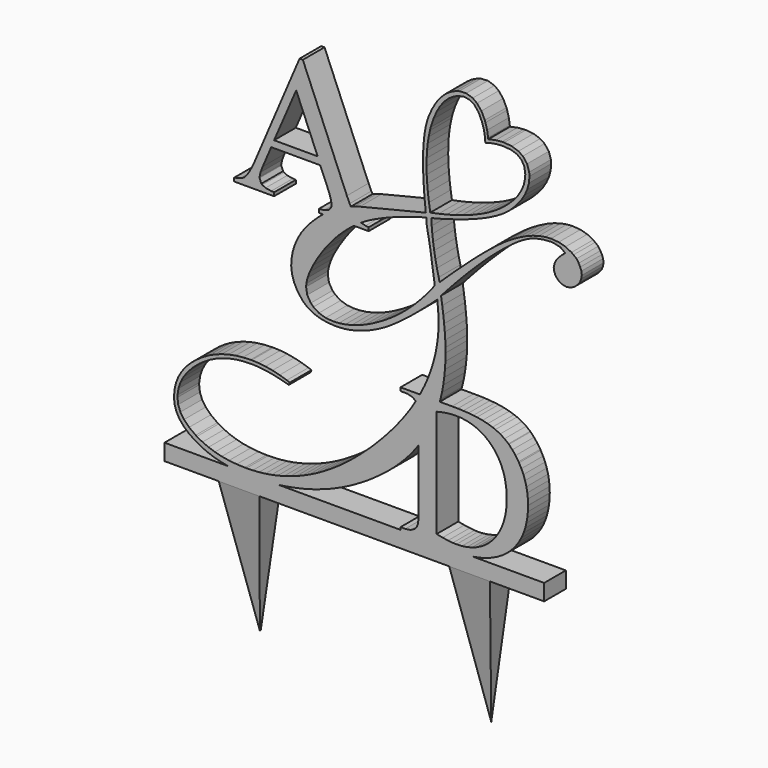
from build123d import *

# Parameters (mm, degrees)
F1_DEPTH = 10
F3_DEPTH = 10
F5_DEPTH = 140.001


# Not quite as in the source:
# - ends of sketch curves that miss each other by under 0.0002 mm in the source are joined


with BuildPart() as f1:
    # F0 (on Front) → F1 (new body)
    with BuildSketch(Plane.XZ):
        Polygon((-10.9298886665, 24.1676968787), (-9.9886611628, 24.5012024907), (-10.4234494528, 25.3038880581), (-11.4401839308, 27.5444704665), (-27.6891162725, 66.3875142995), (-30.1368107855, 55.6929674748), (-22.2288717636, 36.8268846491), (-38.2895193935, 36.8268846491), (-21.26862216, 34.2473902988), (-18.4443582236, 27.5444704665), (-17.8795054363, 26.0946816908), (-17.2769965153, 24.1741824836), (-17.0698830629, 22.7432224485), (-17.2769965153, 21.7076592298), (-18.067790148, 20.8415506343), (-19.5175789237, 20.2202129726), (-19.8564908657, 20.1260706168), (-21.8146462065, 19.9189585121), (-21.8146462065, 18.6386257073), (-20.2368925623, 18.6386257073), (-19.9110483886, 18.9145658222), (-17.7457782476, 20.4961530874), (-15.5428533206, 21.9082857296), (-13.2646134308, 23.13213366), align=None)
        Polygon((-30.1368107855, 55.6929674748), (-27.6891162725, 66.3875142995), (-28.8941354622, 66.3875142995), (-45.2936936863, 27.9586960236), (-45.3690073014, 27.7704126597), (-46.4045705201, 25.5298289035), (-47.3836488644, 23.7034720521), (-48.3250710751, 22.2725120171), (-49.1911783228, 21.2557761913), (-49.3229768124, 21.1428064425), (-50.697451973, 20.4649825587), (-52.9945206036, 19.9189585121), (-52.9945206036, 18.6386257073), (-38.2895193935, 18.6386257073), (-38.2895193935, 19.9189585121), (-39.343911353, 19.9942721272), (-41.4150377904, 20.3331840692), (-42.6577144615, 20.9168655972), (-42.9777976627, 21.1992913169), (-43.6556215466, 22.8373648044), (-43.6556215466, 23.1197905241), (-43.3167096047, 24.7578640116), (-42.5070872313, 26.8666479305), (-39.343911353, 34.2473902988), (-21.26862216, 34.2473902988), (-38.2895193935, 36.8268846491), align=None)
        Polygon((-10.1767511675, -15.6167678171), (-7.6537430394, -15.0330862891), (-16.6349014137, -14.8636303181), (-19.3085381199, -14.6376894728), (-21.7562339807, -13.8657232331), (-23.7897042845, -12.5665630354), (-24.7499538881, -11.6251408247), (-26.0491140858, -9.4410432907), (-26.4821683836, -6.9368625555), (-26.3880260277, -5.788329588), (-25.9549730778, -3.8301728993), (-25.1453507044, -1.6272466246), (-23.9591589076, 0.8392766292), (-22.3964003831, 3.5505708168), (-20.4570724352, 6.487804502), (-19.7604198106, 7.485711587), (-18.0846901895, 9.669809121), (-16.3336469532, 11.7409355585), (-14.5072901019, 13.6990922471), (-12.6056182876, 15.5254490985), (-10.6474629468, 17.2388362011), (-8.885374772, 18.6386257073), (-20.2368925623, 18.6386257073), (-22.0010035668, 17.1446938452), (-24.0533012635, 15.1865371566), (-24.8817523776, 14.3204299088), (-26.7645954511, 12.1551611155), (-28.3650114571, 9.9334061001), (-29.6641730027, 7.655167558), (-30.6620787399, 5.3580989274), (-31.3963874982, 3.0045454224), (-31.8294417959, 0.6133357838), (-31.9800690262, -1.8155313363), (-31.9612402854, -2.0603009224), (-31.6788145657, -4.5268241761), (-30.9256770667, -6.9180351625), (-29.7018291363, -9.2715873197), (-28.0072707745, -11.5309984688), (-27.5177316023, -12.0770238632), (-25.7666883661, -13.5456400319), (-23.6767331879, -14.6753456065), (-21.2666948085, -15.4849679798), (-18.536573228, -15.974507152), (-15.4675397055, -16.1439631229), (-15.0909702821, -16.1439631229), (-12.6432757691, -15.9933358927), align=None)
        Polygon((-9.4443711085, 23.4963599475), (-9.9886611628, 24.5012024907), (-10.9298886665, 24.1676968787), (-13.2646134308, 23.13213366), (-15.5428533206, 21.9082857296), (-17.7457782476, 20.4961530874), (-19.9110483886, 18.9145658222), (-20.2368925623, 18.6386257073), (-8.885374772, 18.6386257073), (-8.6328213837, 18.8392522071), (-6.5240374648, 20.3078697236), (-6.1985443859, 20.5113026795), (-6.4318224604, 20.5779536553), (-7.8627838432, 21.4628896437), (-8.5029502456, 22.1407121798), align=None)
        Polygon((14.6391139914, 29.100744734), (17.8964308778, 30.0421655968), (17.6751323737, 31.5131313185), (-6.6558359543, 25.5610007801), (-8.5386790279, 25.0149753857), (-9.9886611628, 24.5012024907), (-9.4443711085, 23.4963599475), (-8.5029502456, 22.1407121798), (-7.8627838432, 21.4628896437), (-6.4318224604, 20.5779536553), (-6.1985443859, 20.5113026795), (-5.0177624669, 21.2492905864), (-3.1914056155, 22.2660250644), (-1.1767640525, 23.2639321495), (1.0073334815, 24.2618392345), (3.3797143794, 25.2597449718), (5.9215525961, 26.2388233161), (8.6516741767, 27.1990729197), (11.5512517282, 28.1593225233), align=None)
        Polygon((19.3254703004, 30.5748801363), (19.3520434895, 30.3486104282), (19.6851315955, 30.4187336724), (23.0742483192, 31.3036696609), (26.4068801685, 32.2450918716), (29.5512273061, 33.2053414752), (32.4884609913, 34.1655910788), (35.2185839196, 35.1446694231), (37.7604207885, 36.1425751604), (40.0951455527, 37.1593109862), (42.2227582124, 38.1948742049), (44.1432574196, 39.2304374236), (45.8754719151, 40.284829383), (47.4005743059, 41.3580500832), (48.7185645922, 42.4312694356), (50.8838333855, 44.6153669696), (52.6913628439, 46.7994645036), (54.0846667453, 49.0212195191), (55.0825724825, 51.2429731867), (55.6850827513, 53.4835555951), (55.8733661152, 55.7429667443), (55.7792251071, 57.0986131642), (55.0072588674, 59.5274802843), (53.4444989951, 61.5044657137), (51.8064268554, 62.577685066), (46.1578989826, 62.3894017021), (49.0574765341, 62.1446321161), (51.3733725576, 61.3726658764), (53.0114460451, 60.0546769379), (54.0093517824, 58.2283187387), (54.3482637243, 55.8747665816), (54.2352939755, 54.3496628429), (53.7645835441, 52.2032227903), (52.8608188149, 50.0944388714), (51.5804860101, 48.0044836933), (49.8670989075, 45.9521859966), (47.7771437293, 43.9375444335), (45.2729629941, 41.9229028705), (44.2750559091, 41.2450789866), (42.3922141833, 40.040059797), (40.3775726203, 38.9103542224), (38.2123024792, 37.8371335222), (35.9152351964, 36.839227785), (33.4863680763, 35.8789781814), (30.9257024667, 34.9940421929), (28.2144082791, 34.1844198195), (25.3901443427, 33.4124535798), (22.415253176, 32.715802303), (19.3085635199, 32.0756359006), align=None)
        Polygon((19.3085635199, 32.0756359006), (17.8964308778, 30.0421655968), (19.3520435853, 30.3486099733), (19.3254703004, 30.5748801363), align=None)
        Polygon((17.6751323737, 31.5131313185), (17.8964308778, 30.0421655968), (19.3085635199, 32.0756359006), (17.8964308778, 31.5672679877), align=None)
        Polygon((17.8964308778, 31.5672679877), (19.3085635199, 32.0756359006), (18.8232483473, 35.2102505875), (18.4368979524, 38.2410969438), (18.1737322688, 41.1571122421), (17.9853100817, 43.980424633), (17.9200726059, 46.688904618), (17.9714412383, 49.3001948754), (18.1041319702, 51.801140895), (18.3534301582, 54.204897187), (18.7082690314, 56.4872438179), (19.1797140128, 58.6723993735), (19.466277473, 59.8442115114), (20.4793176362, 62.8943677724), (21.6370452829, 65.5563891538), (22.9615912596, 67.8787155224), (24.4726886794, 69.8084188435), (26.1329617509, 71.3918485489), (27.97978357, 72.5826565544), (29.3693621572, 73.221225816), (31.6930511498, 73.7257511562), (33.7529356025, 73.4286411752), (35.5600822863, 72.354118502), (37.0923590069, 70.453740574), (38.3345262104, 67.8222993858), (36.5379354821, 73.1808040004), (34.9601409209, 74.3408255997), (32.5618149078, 75.1145938456), (30.0162918109, 74.9895383904), (28.7131515651, 74.604227148), (26.6618229353, 73.638597134), (24.7728258152, 72.2914081477), (23.0395816019, 70.5803055631), (21.444447617, 68.4987107771), (20.0292878202, 66.0421356218), (18.7390837414, 63.2503536218), (18.1938346788, 61.6405084197), (17.7209286841, 59.8365964516), (17.3380084357, 57.845193625), (17.0384980261, 55.6839426181), (16.8113320322, 53.3286261931), (16.6741517845, 50.7858175617), (16.6269586308, 48.0555194196), (16.6631739682, 45.1553730972), (16.7893763996, 42.0677372641), (16.9879232467, 38.7860333172), (17.2698785849, 35.334482538), (17.6244923758, 31.8497341414), (17.6751323737, 31.5131313185), align=None)
        Polygon((46.1578989826, 62.3894017021), (51.8064268554, 62.577685066), (49.3963884761, 63.4061361801), (46.5344670582, 63.6697345069), (45.7625021663, 63.6509057662), (43.4466061428, 63.4437936616), (41.1307087715, 62.9542544894), (40.6390589473, 62.8273781589), (40.6869516082, 61.630595364), (41.3943070983, 61.8433776556), (43.7478606032, 62.2576018648), align=None)
        Polygon((36.5379354821, 73.1808040004), (38.3345262104, 67.8222993858), (39.0528487343, 65.5180267738), (39.486804709, 63.1680314561), (39.6073046063, 61.3058231729), (40.686951551, 61.6305955543), (40.639059768, 62.8273781917), (40.6197840854, 63.309063711), (40.2695506387, 65.650081345), (39.6546824083, 67.8924468904), (39.4026791893, 68.6223645222), (38.1560238179, 71.2119444463), align=None)
        Polygon((16.1642163823, -26.9138235628), (15.4680634141, -28.2097382624), (22.7963671558, -28.2097382624), (23.0365921855, -27.3657052535), (23.6202723657, -24.880353259), (24.090984145, -22.3385150423), (24.4487234798, -19.759020692), (24.7123218066, -17.1042127265), (24.8817777776, -14.4117486274), (24.938262652, -11.6627983062), (24.9006065183, -9.8740975885), (24.8252915554, -7.4828879498), (24.6558369322, -4.9598784739), (24.4110673462, -2.3238992492), (24.1098115379, 0.4438798128), (23.7144147216, 3.3434573644), (23.2625330309, 6.3748347532), (24.9570913927, 8.2576764789), (26.8964193406, 10.4041178793), (22.754165118, 10.5924012432), (22.3964257831, 12.0798475004), (21.7562593807, 14.8476252146), (21.2102339864, 17.577748143), (20.7395235549, 20.2325561084), (20.3629554793, 22.8497065924), (20.0617010189, 25.4292009427), (19.8357588257, 27.9522104187), (19.6851315955, 30.4187336724), (19.3520435853, 30.3486099733), (17.8964308778, 30.0421655968), (18.0282307151, 27.0861031709), (18.1788579453, 26.5212503837), (18.630739636, 24.2430104938), (19.3085635199, 20.3078697236), (20.9654644003, 8.9355003628), (19.7416178177, 7.3539117497), (17.9529171, 5.1698142157), (21.8692291295, 4.6991037843), (22.0951699748, 2.5714924725), (22.3022834273, -0.1586291081), (22.3775970424, -2.4556977387), (22.3399395609, -4.0561137447), (22.2269698121, -6.3531823753), (21.9822002261, -8.6502496581), (21.6244595434, -10.9284895479), (21.1725778527, -13.2255568307), (20.6077250654, -15.5037967205), (19.9299011816, -17.8008653511), (19.1579362897, -20.0791038932), (18.2730003012, -22.357343783), (17.2750932161, -24.6355836729), align=None)
        Polygon((19.2897347792, 2.3455516271), (21.8692291295, 4.6991037843), (17.9529171, 5.1698142157), (16.1265589008, 3.117516519), (14.2437171751, 1.1405310896), (12.3420453608, -0.7234818954), (10.38389002, -2.4745264794), (8.3880758498, -4.1314273598), (6.3546068939, -5.6753584914), (4.2834791086, -7.1251472672), (2.1746951897, -8.4619649464), (0.4989655686, -9.4598720314), (-2.1370136561, -10.8908320664), (-4.7165080064, -12.1146799969), (-7.2395174823, -13.0937583412), (-9.6872119954, -13.8657232331), (-12.0595942411, -14.4305760204), (-14.3754902646, -14.7506592216), (-16.6349014137, -14.8636303181), (-7.6537430394, -15.0330862891), (-5.1119048227, -14.2234639157), (-2.5135817317, -13.187900697), (0.122397493, -11.9263952852), (0.6119366652, -11.6816256991), (2.2876662863, -10.7590335769), (4.0575382633, -9.666984136), (5.9215525961, -8.4243088127), (7.8985366777, -7.0310049113), (9.9696644629, -5.4682463868), (12.1537619969, -3.7548592842), (14.432000539, -1.8720162107), (16.8043827847, 0.1614540931), align=None)
        Polygon((22.754165118, 10.5924012432), (26.8964193406, 10.4041178793), (28.8169185478, 12.4752443167), (30.7185890143, 14.4898858798), (32.6014320878, 16.4292138277), (34.4654464206, 18.3120555534), (36.291803272, 20.1195850119), (38.1181614712, 21.8706282481), (39.906860841, 23.5651866099), (41.676732818, 25.1656026159), (42.2039294716, 25.6363143952), (44.8587374371, 27.9145529372), (47.3064332979, 29.9103671073), (49.5281869656, 31.6237528621), (51.5239997879, 33.0358855042), (53.2938717648, 34.1655910788), (54.8566316372, 35.0128695858), (56.0804795676, 35.5588949802), (58.6223164365, 36.4061734872), (61.1829833939, 36.8957126593), (63.8001338778, 37.0651686303), (69.1850634238, 37.1969671198), (66.6620552957, 37.8747910037), (63.8001338778, 38.100731849), (61.6725212182, 37.9501046188), (59.3754539354, 37.5358790617), (56.9654155561, 36.8203990442), (54.4612348209, 35.8224919592), (51.8252555961, 34.5421591544), (49.0951326678, 32.9794006298), (47.7771437293, 32.132120775), (46.3085262128, 31.13421369), (44.7269389476, 29.9856807225), (43.0323805857, 28.6865191769), (41.2248511273, 27.2555591419), (39.3231806608, 25.6739705288), (37.2897103571, 23.9605834263), (35.1432689567, 22.0965704412), (32.9026865483, 20.0819288782), (30.5303056504, 17.9166587371), (28.0449536559, 15.6195914543), (25.4654593056, 13.1718955935), align=None)
        Polygon((69.1850634238, 37.1969671198), (63.8001338778, 37.0651686303), (64.5909275105, 37.0275111489), (67.2645642166, 36.4250022279), (69.0532649343, 35.1446694231), (69.0344361936, 35.0505270673), (67.9642696041, 34.1886222543), (67.0009658898, 33.2241702159), (66.247446964, 32.4437330646), (65.6371720299, 31.5799359429), (65.1351333773, 30.4364666532), (64.8356970966, 29.1384008676), (64.9674969339, 27.8957255443), (65.4550750597, 26.7201368759), (66.2290009979, 25.6927992696), (67.1139369864, 24.977319252), (68.2955651385, 24.5026826845), (69.5616328472, 24.2806666275), (71.1620488532, 24.563093695), (72.3996308472, 25.2280824967), (73.4026312616, 26.0693673451), (74.5511655769, 27.500328728), (74.971341663, 28.6815458016), (75.1913319793, 29.9103671073), (75.0407047491, 31.2283560458), (74.581185086, 32.3683803633), (74.042797664, 33.4501110613), (73.2342090519, 34.6332703121), (72.1222984568, 35.5400662394), (71.3691609579, 36.086090286), align=None)
        Polygon((14.9403684519, -29.1920621048), (13.9460917161, -30.8965359279), (14.0773234016, -30.9963460652), (14.6045200552, -32.0507380246), (14.9246032564, -33.877094876), (15.0375730052, -36.4565892263), (15.0375730052, -44.7636998826), (16.013589152, -43.3322105276), (17.3315780905, -41.204597868), (18.5554260209, -39.0393290747), (19.6663028547, -36.7987466663), (20.6642099398, -34.5205067764), (21.5491459283, -32.1857820122), (21.6463504816, -31.8941683522), (21.6463504816, -31.7871396978), (21.6850938894, -31.777938129), (22.3399395609, -29.8134011143), (22.7963671558, -28.2097382624), (15.4680634141, -28.2097382624), align=None)
        Polygon((12.7405057224, -29.9796102394), (13.9460917161, -30.8965359279), (14.9403684519, -29.1920621048), (15.4680634141, -28.2097382624), (8.3346545207, -28.2097382624), (8.3346545207, -29.4524149336), (10.085697757, -29.4524149336), (10.8953201303, -29.4900710672), align=None)
        Polygon((-48.4737696061, -72.9304963116), (-60.4674779763, -73.2317507721), (-58.0009533748, -73.9095746559), (-55.3838028908, -74.4367699617), (-52.6536799624, -74.8133380373), (-49.7917598924, -75.0392802305), (-46.798039985, -75.1145938456), (-45.5553646617, -75.0957651049), (-42.9005553484, -75.0204514898), (-40.2645761237, -74.8509955188), (-37.6474256397, -74.6062259327), (-35.0679312894, -74.2861427315), (-32.507264332, -73.8530884337), (-29.9654274631, -73.3635492616), (-27.4612467279, -72.7798690814), (-24.9758947334, -72.1208739382), (-22.5281988726, -71.3677364392), (-20.0993317525, -70.5204579322), (-17.6892933732, -69.616693203), (-15.3169124753, -68.618786118), (-12.9445302296, -67.5267380249), (-10.628634206, -66.3593749688), (-8.3127368347, -65.0978709048), (-6.0533270334, -63.7610532256), (-3.7939158843, -62.3489205835), (-1.5721608688, -60.8426469333), (0.6307654059, -59.2610583203), (2.8148615921, -57.5853286991), (3.8315974179, -56.756877585), (5.8838951146, -55.0058343488), (7.8420518033, -53.1794774975), (9.6872373954, -51.3154631646), (11.4382819794, -49.3949639575), (13.0575253783, -47.4368072688), (14.6014565099, -45.403336965), (15.0375730052, -44.7636998826), (15.0375730052, -36.4565892263), (14.9246032564, -33.877094876), (14.6045200552, -32.0507380246), (14.0773234016, -30.9963460652), (13.9460917161, -30.8965359279), (13.6223781656, -31.4514732539), (12.1914181306, -33.7297131438), (10.647486999, -35.9891242929), (8.9905861186, -38.2485354421), (7.2207141416, -40.5079465912), (5.3566998088, -42.7673577403), (3.3797143794, -45.0267688894), (1.2897592013, -47.2861800386), (-0.8943369849, -49.526762447), (-2.9089798958, -51.5037478763), (-5.1683896971, -53.5937030545), (-7.4089734533, -55.5706871361), (-9.6683846024, -57.4535302096), (-11.9089670108, -59.2234021866), (-14.16837816, -60.880303067), (-16.4277893091, -62.4242341986), (-18.7060291989, -63.8740229744), (-20.9654403481, -65.2108420013), (-23.2436788901, -66.4535173247), (-25.52191878, -67.5832228992), (-27.8001586698, -68.5999573772), (-30.0783972119, -69.5037221064), (-32.3566371018, -70.3133444798), (-34.6537057323, -71.0099971044), (-36.9507730151, -71.5936772846), (-39.2478416457, -72.0832164568), (-41.5449089285, -72.4597858802), (-43.8419775591, -72.7233828592), (-46.1578735826, -72.8740100894), align=None)
        Polygon((27.3137070952, -28.2097382624), (22.7963671558, -28.2097382624), (22.3399395609, -29.8134011143), (21.6850938894, -31.777938129), (23.1526254796, -31.4293990152), (25.1107808204, -31.0716596803), (26.9747951532, -30.8645462279), (28.7258397373, -30.7892326128), (43.29904111, -30.5444630267), (42.2069916691, -30.1302374696), (40.4559484329, -29.5653846824), (38.5542779664, -29.1135029917), (36.5019789219, -28.755762309), (35.1651612427, -28.5863076858), (33.3952892658, -28.4168517149), (31.4747900586, -28.3038806183), (29.4601484955, -28.2285670032), align=None)
        Polygon((28.9706093234, -72.4565390343), (13.6066129702, -72.475367775), (12.10033932, -73.3038188891), (10.085697757, -73.5862446089), (8.3346545207, -73.5862446089), (8.3346545207, -74.8854061544), (29.177721428, -74.8854061544), (29.2906925246, -74.8854061544), (31.3994750956, -74.82892128), (33.4141166587, -74.6782940498), (35.3346172137, -74.4335244637), (37.160974065, -74.0946125218), (38.9120173013, -73.661558224), (40.5877482702, -73.1343629182), (40.6254044038, -73.1155341774), (42.5082474774, -72.3623980263), (44.2592907136, -71.4962894307), (45.8785354603, -70.5172110864), (47.3659803698, -69.4251629933), (48.7404555304, -68.2201438036), (49.7195338747, -67.2222367185), (50.9245530644, -65.7724479428), (51.9977737646, -64.2096894182), (52.9203672345, -62.5527871901), (53.6923321264, -60.7640864724), (53.7299882601, -60.6887728572), (54.3136697881, -58.937729621), (54.7655528266, -57.1302015104), (55.1044634208, -55.2473584368), (55.2927481324, -53.3080304889), (55.3680617476, -51.3122176666), (55.3680617476, -51.19924657), (55.2927481324, -49.184605007), (55.0856360278, -47.2452770591), (54.7467240859, -45.3624339855), (54.2571849137, -43.5360771342), (53.654674645, -41.7850338979), (52.9015384938, -40.1093042768), (52.0354312461, -38.4900595301), (51.8659752751, -38.2076324625), (50.7550970935, -36.5507315822), (49.5689066445, -35.0632853249), (48.2885738397, -33.7452963865), (48.1379466095, -33.5946678084), (46.6881578337, -32.4273061002), (45.068913087, -31.4105716222), (43.29904111, -30.5444630267), (28.7258397373, -30.7892326128), (28.8576382268, -30.7892326128), (30.8346223084, -30.8833749686), (32.7362941226, -31.1658020362), (34.562650974, -31.6176837269), (36.2948668173, -32.2390213885), (37.7069981116, -32.9168452724), (39.3450715991, -33.9147510096), (40.8325165085, -35.0821140657), (42.2069916691, -36.4189317449), (42.2258204098, -36.4189317449), (43.3931834659, -37.8498931277), (44.4475754253, -39.4126516522), (45.3513388067, -41.1072100141), (46.1233050464, -42.9523956062), (46.4622169884, -44.0067875656), (46.9140986791, -45.7766595426), (47.2341818803, -47.6406738754), (47.4412953327, -49.598830564), (47.4977802071, -51.6511282607), (47.4789514663, -52.8373200575), (47.3283242361, -54.8331328798), (47.0647259093, -56.7348033463), (46.6505003523, -58.5423328047), (46.1233050464, -60.274548648), (46.1044763057, -60.2933760409), (45.3325114138, -62.1573903737), (44.4475754253, -63.8519487356), (43.4120108588, -65.4147086079), (42.2446491506, -66.845668643), (41.1714284504, -67.9188893431), (39.7028109339, -69.1239085328), (38.1023949279, -70.1594717515), (36.3890091731, -71.0067502585), (34.6756220706, -71.628089268), (32.8492652192, -72.0987996995), (30.9475934049, -72.3812254192), align=None)
        Polygon((16.013589152, -43.3322105276), (15.0375730052, -44.7636998826), (15.0375730052, -66.6385565383), (14.9810881308, -68.5402270048), (14.7363185447, -70.5172110864), (14.284436854, -71.7222316239), (13.6066129702, -72.475367775), (28.9706093234, -72.4565390343), (27.6337902964, -72.4188829007), (25.8450895787, -72.2494269297), (23.8492767564, -71.9481724692), (21.6463504816, -71.5151181714), (21.6463504816, -31.8941683522), (21.5491459283, -32.1857820122), (20.6642099398, -34.5205067764), (19.6663028547, -36.7987466663), (18.5554260209, -39.0393290747), (17.3315780905, -41.204597868), align=None)
        Polygon((-46.798039985, -38.5309611618), (-55.0637196896, -38.1920505677), (-57.5679004248, -38.8698731037), (-59.9779388042, -39.7548090922), (-62.2938348277, -40.8092010516), (-64.5155884954, -42.0707064635), (-66.6243724142, -43.5204952393), (-66.6620298957, -43.5393226322), (-68.9214410448, -45.3845082243), (-70.841940252, -47.3238361722), (-72.4046987766, -49.3761352167), (-73.628546707, -51.5225752693), (-74.4946553025, -53.7819864184), (-75.0218506084, -56.1543686641), (-75.1913065793, -58.6020631771), (-75.0030218676, -60.710847096), (-74.3440267245, -62.9137733708), (-73.2143211499, -64.9660724153), (-71.6139051439, -66.9054003632), (-69.5427787065, -68.7129284738), (-67.0009418376, -70.369830702), (-65.0239564082, -71.4430500544), (-62.8022027406, -72.4221283987), (-60.4674779763, -73.2317507721), (-48.4737696061, -72.9304963116), (-49.1139360085, -72.9304963116), (-52.0888271752, -72.817525215), (-54.9130911116, -72.5350994953), (-57.5867278177, -72.0832164568), (-60.1097372937, -71.4618787951), (-62.4821195394, -70.6710851625), (-64.6850444663, -69.7108355589), (-66.7561722516, -68.5811299843), (-67.1892252015, -68.3175316575), (-69.6180923216, -66.5476596805), (-71.5009353952, -64.6459892141), (-72.8377530743, -62.631347651), (-73.6473754477, -60.5037349914), (-73.9109737745, -58.2254951015), (-73.8921450338, -57.4723589504), (-73.5532330919, -55.2129478012), (-72.8189243336, -52.9911927858), (-71.6892187591, -50.8447527332), (-70.1452889752, -48.7359688143), (-68.2059610273, -46.6648423769), (-65.8524075223, -44.6690282068), (-64.2331627756, -43.5204952393), (-62.0490652416, -42.1836762123), (-59.751996611, -41.0727993785), (-57.3607869724, -40.1502059085), (-54.8566062372, -39.434725891), (-52.2771118869, -38.9263593259), (-49.5846477877, -38.6251035176), align=None)
        Polygon((-52.4653965985, -37.6836826548), (-55.0637196896, -38.1920505677), (-46.798039985, -38.5309611618), (-46.044902486, -38.5309611618), (-43.597207973, -38.6627609991), (-41.0741984971, -38.9640154596), (-38.4382192723, -39.434725891), (-35.7080976918, -40.0560649005), (-32.8650050147, -40.8280297924), (-32.4884369391, -39.9430938039), (-33.5993137729, -39.5476969876), (-36.2541217383, -38.7192458735), (-38.8901009631, -38.0790794711), (-41.4695953134, -37.6083690397), (-44.030260923, -37.3447707128), (-46.5532703989, -37.250628357), (-46.967495956, -37.250628357), (-49.7729311516, -37.3824281943), align=None)
        Polygon((-4.5866368683, 20.0507570016), (-6.1985443859, 20.5113026795), (-6.5240374648, 20.3078697236), (-8.6328213837, 18.8392522071), (-8.885374772, 18.6386257073), (-3.4192751601, 18.6386257073), (-3.4192751601, 19.9189585121), align=None)
    extrude(amount=F1_DEPTH)

    # F2 (on face) → F3 (join, through all)
    with BuildSketch(Plane.XZ.offset(10)):
        Polygon((-55.0012434608, -74.489536695), (-78.7086935341, -74.489536695), (-78.7086935341, -80.489536695), (-58.7086935341, -80.489536695), (-43.7086935341, -80.489536695), (26.2913064659, -80.489536695), (41.2913064659, -80.489536695), (61.2913064659, -80.489536695), (61.2913064659, -74.489536695), (34.8951364635, -74.489536695), (33.4141166587, -74.6782940498), (31.3994750956, -74.82892128), (29.2906925246, -74.8854061544), (8.3346545207, -74.8854061544), (8.3346545207, -74.489536695), (-36.7070475497, -74.489536695), (-37.6474256397, -74.6062259327), (-40.2645761237, -74.8509955188), (-42.9005553484, -75.0204514898), (-45.5553646617, -75.0957651049), (-46.798039985, -75.1145938456), (-49.7917598924, -75.0392802305), (-52.6536799624, -74.8133380373), align=None)
        Polygon((-43.7086935341, -80.489536695), (-58.7086935341, -80.489536695), (-51.2086935341, -130.489536695), align=None)
        Polygon((41.2913064659, -80.489536695), (26.2913064659, -80.489536695), (33.7913064659, -132.6214164495), align=None)
    extrude(amount=-F3_DEPTH)

    # F4 (on face) → F5 (cut, through all)
    with BuildSketch(Plane.YZ.offset(61.2913064659)):
        Polygon((-9.9999999999, -132.6214164495), (2e-10, -132.6214164495), (-9.9999999999, -80.489536695), align=None)
    extrude(amount=-F5_DEPTH, mode=Mode.SUBTRACT)


solid = f1.part
